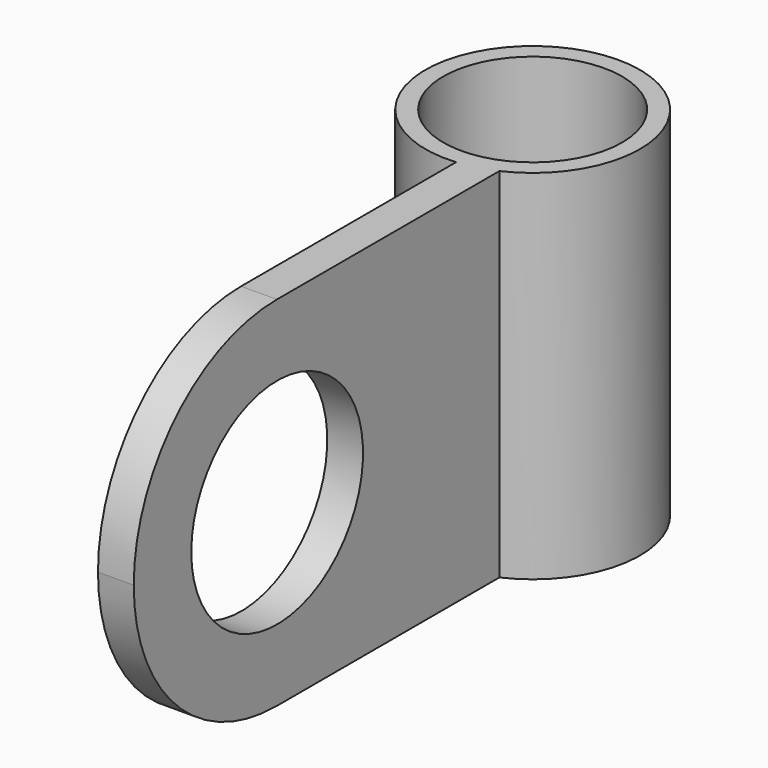
from build123d import *

# Parameters (mm, degrees)
F0_R     = 6
F0_R_2   = 5
F1_DEPTH = 20
F3_DEPTH = 20
F4_R     = 6
F5_DEPTH = 5.501
F6_R     = 9.99999


# Not quite as in the source:
# - a fillet or chamfer is up to 0.001 mm smaller than in the source, because OpenCascade refuses the exact size


with BuildPart() as f1:
    # F0 (on Top) → F1 (new body)
    with BuildSketch(Plane.XY):
        Circle(F0_R)
        Circle(F0_R_2, mode=Mode.SUBTRACT)
    extrude(amount=F1_DEPTH)

    # F2 (on face) → F3 (join)
    with BuildSketch(Plane.XY.offset(20)):
        with BuildLine():
            Line((0.5, -6), (0.5, -31))
            Line((0.5, -31), (2.5, -31))
            Line((2.5, -31), (2.5, -6))
            Line((2.5, -6), (2.5, -5.4543560573))
            ThreePointArc((2.5, -5.4543560573), (1.52277609, -5.8035465863), (0.5, -5.9791303716))
            Line((0.5, -5.9791303716), (0.5, -6))
        make_face()
    extrude(amount=-F3_DEPTH)

    # F4 (on face) → F5 (cut, through all)
    with BuildSketch(Plane(origin=(0.5, 0, 0), x_dir=(0, -1, 0), z_dir=(-1, 0, 0))):
        with Locations((20.9791303716, 10)):
            Circle(F4_R)
    extrude(amount=-F5_DEPTH, mode=Mode.SUBTRACT)

    # F6 (radius 10 in the source; OpenCascade refuses exactly that, so slightly less here)
    f6_edges = [f1.edges().sort_by_distance(p)[0] for p in [
        (1.5, -31, 20),
        (1.5, -31, 0),
    ]]
    fillet(f6_edges, radius=F6_R)


solid = f1.part
